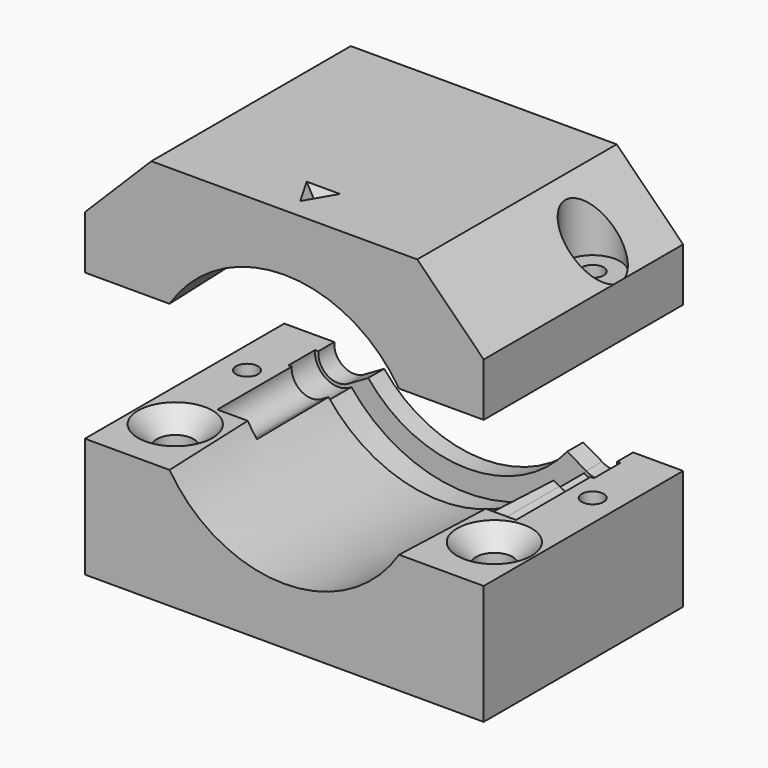
from build123d import *

# Parameters (mm, degrees)
F1_W              = 60
F1_H              = 18
F2_DEPTH          = 29.5
F2_DEPTH_BACK     = 8
F3_DEPTH          = 5
F4_R              = 19.25
F5_DEPTH          = 25
F6_R              = 21.5
F7_DEPTH          = 30
F7_TAPER          = 2
F9_DEPTH          = 14
F12_SIZE          = 10
F14_D             = 5.5
F14_DEPTH         = 40
F14_CSINK_D       = 11.2
F14_CSINK_ANGLE   = 90
F14_TIP           = 1.6523667023
F16_D             = 3.3
F16_DEPTH         = 58
F16_CBORE_D       = 8.25
F16_CBORE_DEPTH   = 10
F16_TIP           = 0.9914200214
F16_2_D           = 3.3
F16_2_DEPTH       = 58
F16_2_CBORE_D     = 8.25
F16_2_CBORE_DEPTH = 10
F16_2_TIP         = 0.9914200214


# Not quite as in the source:
# - an extrude whose draft closes it to a point is written as a loft to that point


with BuildPart() as f2:
    # F1 (on Front) → F2 (new body, two sides)
    with BuildSketch(Plane.XZ) as f2_sk:
        with Locations((0, -20)):
            Rectangle(F1_W, F1_H)
    extrude(amount=F2_DEPTH)
    extrude(f2_sk.sketch, amount=-F2_DEPTH_BACK)


with BuildPart() as f2b:
    # F1 (on Front) → F2, piece 2 (new body, two sides)
    with BuildSketch(Plane.XZ) as f2_2_sk:
        with Locations((0, 20)):
            Rectangle(F1_W, F1_H)
    extrude(amount=F2_DEPTH)
    extrude(f2_2_sk.sketch, amount=-F2_DEPTH_BACK)


with BuildPart() as f3_tool:
    # F0 (on Front) → F3 (new body)
    with BuildSketch(Plane.XZ):
        with BuildLine():
            Line((-5, 20.0000014156), (-10.3077613174, 20.0000014156))
            ThreePointArc((-10.3077613174, 20.0000014156), (-21.0296949807, 8.0001205627), (-20.9945189859, -8.0919819915))
            ThreePointArc((-20.9945189859, -8.0919819915), (-22.5166604984, -13), (-17.5051214646, -14.1357957862))
            ThreePointArc((-17.5051214646, -14.1357957862), (0, -22.5), (17.5051214646, -14.1357957862))
            ThreePointArc((17.5051214646, -14.1357957862), (22.5166604984, -13), (20.9945189859, -8.0919819915))
            ThreePointArc((20.9945189859, -8.0919819915), (21.0296949807, 8.0001205627), (10.3077613174, 20.0000014156))
            Line((10.3077613174, 20.0000014156), (5, 20.0000014156))
            Line((5, 20.0000014156), (5, 24.9999985844))
            Line((5, 24.9999985844), (-5, 24.9999985844))
            Line((-5, 24.9999985844), (-5, 20.0000014156))
        make_face()
    extrude(amount=-F3_DEPTH)


with BuildPart() as f2_1:
    add(f2.part)

    # F3: cut by f3_tool
    add(f3_tool.part, mode=Mode.SUBTRACT)


with BuildPart() as f2b_1:
    add(f2b.part)

    # F3: cut by f3_tool
    add(f3_tool.part, mode=Mode.SUBTRACT)


with BuildPart() as f5_tool:
    # F4 (on Front) → F5 (new body)
    with BuildSketch(Plane.XZ):
        Circle(F4_R)
    extrude(amount=-F5_DEPTH)


with BuildPart() as f2_2:
    add(f2_1.part)

    # F5: cut by f5_tool
    add(f5_tool.part, mode=Mode.SUBTRACT)


with BuildPart() as f2b_2:
    add(f2b_1.part)

    # F5: cut by f5_tool
    add(f5_tool.part, mode=Mode.SUBTRACT)


with BuildPart() as f7_tool:
    # F6 (on Front) → F7 (new body)
    with BuildSketch(Plane.XZ):
        Circle(F6_R)
    extrude(amount=F7_DEPTH, taper=F7_TAPER)


with BuildPart() as f2_3:
    add(f2_2.part)

    # F7: cut by f7_tool
    add(f7_tool.part, mode=Mode.SUBTRACT)


with BuildPart() as f2b_3:
    add(f2b_2.part)

    # F7: cut by f7_tool
    add(f7_tool.part, mode=Mode.SUBTRACT)


with BuildPart() as f9_tool:
    # F8 (on Front) → F9 (new body, symmetric)
    with BuildSketch(Plane.XZ):
        with BuildLine():
            ThreePointArc((2.9933259094, 22.3), (0, 25.5), (-2.9933259094, 22.3))
            Line((-2.9933259094, 22.3), (-2.9933259094, 16.3133481812))
            Line((-2.9933259094, 16.3133481812), (2.9933259094, 16.3133481812))
            Line((2.9933259094, 16.3133481812), (2.9933259094, 22.3))
        make_face()
        with BuildLine():
            ThreePointArc((17.8157035497, -13.7422962794), (22.0836477965, -12.75), (20.8090294591, -8.5577037206))
            Line((20.8090294591, -8.5577037206), (15.6244369004, -5.5643778112))
            Line((15.6244369004, -5.5643778112), (12.631110991, -10.7489703699))
            Line((12.631110991, -10.7489703699), (17.8157035497, -13.7422962794))
        make_face()
        with BuildLine():
            ThreePointArc((-20.8090294591, -8.5577037206), (-22.0836477965, -12.75), (-17.8157035497, -13.7422962794))
            Line((-17.8157035497, -13.7422962794), (-12.631110991, -10.7489703699))
            Line((-12.631110991, -10.7489703699), (-15.6244369004, -5.5643778112))
            Line((-15.6244369004, -5.5643778112), (-20.8090294591, -8.5577037206))
        make_face()
    extrude(amount=F9_DEPTH, both=True)


with BuildPart() as f2_4:
    add(f2_3.part)

    # F9: cut by f9_tool
    add(f9_tool.part, mode=Mode.SUBTRACT)

    # F14
    with Locations(Plane.XY.offset(-11)):
        with Locations((-24, -20), (24, -20)):
            CounterSinkHole(F14_D / 2, F14_CSINK_D / 2, depth=F14_DEPTH, counter_sink_angle=F14_CSINK_ANGLE)
            with Locations((0, 0, -(F14_DEPTH + F14_TIP / 2))):  # 118° drill point
                Cone(0, F14_D / 2, F14_TIP, mode=Mode.SUBTRACT)

    # F16
    with Locations(Plane.XY.offset(29)):
        with Locations((-26, -4), (26, -4)):
            CounterBoreHole(F16_D / 2, F16_CBORE_D / 2, F16_CBORE_DEPTH, depth=F16_DEPTH)
            with Locations((0, 0, -(F16_DEPTH + F16_TIP / 2))):  # 118° drill point
                Cone(0, F16_D / 2, F16_TIP, mode=Mode.SUBTRACT)


with BuildPart() as f2b_4:
    add(f2b_3.part)

    # F9: cut by f9_tool
    add(f9_tool.part, mode=Mode.SUBTRACT)

    # F10 (on face) → F11 section 0
    with BuildSketch(Plane.XY.offset(29), mode=Mode.PRIVATE) as f11_s0:
        Polygon((-2.5, -22.1698729811), (0, -26.5), (2.5, -22.1698729811), align=None)
    loft([f11_s0.sketch, Vertex(0, -23.6132486541, 27.556624327)], ruled=True, mode=Mode.SUBTRACT)

    # F12
    f12_edges = [f2b_4.edges().sort_by_distance(p)[0] for p in [
        (30, -10.75, 29),
        (-30, -10.75, 29),
    ]]
    chamfer(f12_edges, length=F12_SIZE)

    # F16#2
    with Locations(Plane.XY.offset(29)):
        with Locations((-26, -4), (26, -4)):
            CounterBoreHole(F16_2_D / 2, F16_2_CBORE_D / 2, F16_2_CBORE_DEPTH, depth=F16_2_DEPTH)
            with Locations((0, 0, -(F16_2_DEPTH + F16_2_TIP / 2))):  # 118° drill point
                Cone(0, F16_2_D / 2, F16_2_TIP, mode=Mode.SUBTRACT)


solid = Compound([f2_4.part, f2b_4.part])
